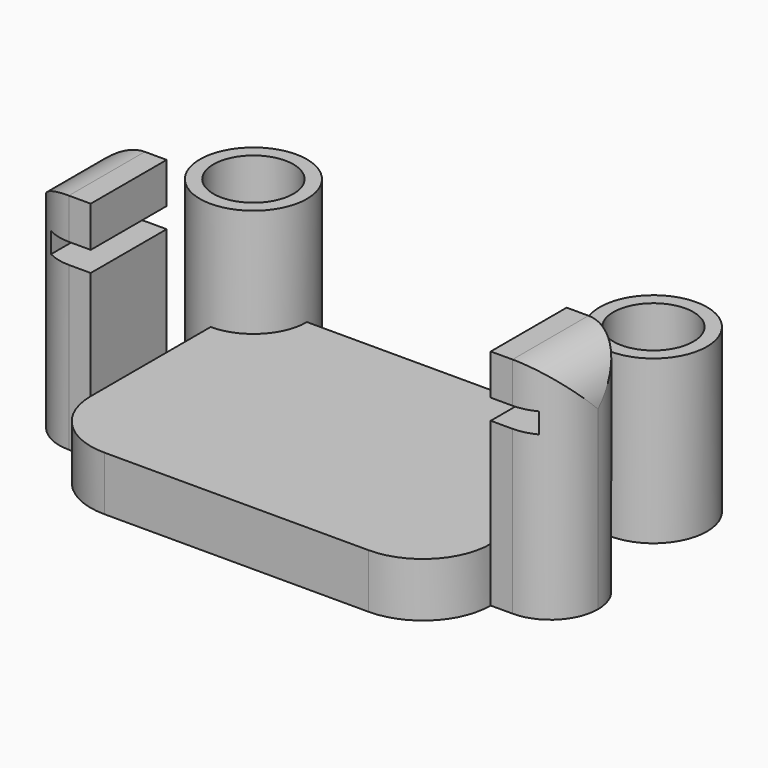
from build123d import *

# Parameters (mm, degrees)
F0_R         = 3.95
F0_R_2       = 2.95
F1_DEPTH     = 12
F3_DEPTH     = 4
F5_R         = 5
F6_W         = 3
F6_H         = 7
F6_W_2       = 2.1112600537
F7_DEPTH     = 16.5
F8_W         = 3.25
F8_H         = 1.5
F9_DEPTH     = 7
F10_T1_DEPTH = 34
F10_T3_DEPTH = 24.5


# Not quite as in the source:
# - a fillet or chamfer that OpenCascade refuses, or shapes differently, is made with other operations: its cross-section is extruded or revolved along the edge and cut away or added


with BuildPart() as f1:
    # F0 (on Top) → F1 (new body)
    with BuildSketch(Plane.XY):
        Circle(F0_R)
        Circle(F0_R_2, mode=Mode.SUBTRACT)
    extrude(amount=F1_DEPTH)


with BuildPart() as f1b:
    # F0 (on Top) → F1, piece 2 (new body)
    with BuildSketch(Plane.XY):
        with Locations((29.5, 0)):
            Circle(F0_R)
        with Locations((29.5, 0)):
            Circle(F0_R_2, mode=Mode.SUBTRACT)
    extrude(amount=F1_DEPTH)


with BuildPart() as f3:
    # F2 (on face) → F3 (new body)
    with BuildSketch(Plane(origin=(0, 0, 0), x_dir=(1, 0, 0), z_dir=(0, 0, -1))):
        with BuildLine():
            ThreePointArc((0, 3.95), (2.7930717857, 2.7930717857), (3.95, 0))
            Line((3.95, 0), (25.55, 0))
            ThreePointArc((25.55, 0), (26.7069282143, 2.7930717857), (29.5, 3.95))
            Line((29.5, 3.95), (29.5, 20))
            Line((29.5, 20), (0, 20))
            Line((0, 20), (0, 3.95))
        make_face()
    extrude(amount=-F3_DEPTH)

    # F4: union F1, F1b
    add(f1.part)
    add(f1b.part)

    # F5
    f5_edges = [f3.edges().sort_by_distance(p)[0] for p in [
        (0, -20, 2),
        (29.5, -20, 2),
    ]]
    fillet(f5_edges, radius=F5_R)

    # F6 (on face) → F7 (join)
    with BuildSketch(Plane(origin=(0, 0, 0), x_dir=(1, 0, 0), z_dir=(0, 0, -1))):
        with Locations((-3.6112600537, 11.5)):
            Rectangle(F6_W, F6_H)
        with Locations((-1.0556300269, 11.5)):
            Rectangle(F6_W_2, F6_H)
        with Locations((30.5556300269, 11.5)):
            Rectangle(F6_W_2, F6_H)
        with Locations((33.1112600537, 11.5)):
            Rectangle(F6_W, F6_H)
    extrude(amount=-F7_DEPTH)

    # F8 (on face) → F9 (cut, through all)
    with BuildSketch(Plane.XZ.offset(15)):
        with Locations((-1.625, 12.75)):
            Rectangle(F8_W, F8_H)
        with Locations((31.125, 12.75)):
            Rectangle(F8_W, F8_H)
    extrude(amount=-F9_DEPTH, mode=Mode.SUBTRACT)

    # F10: fillet of radius 3.5 on 6 edges, made by hand

    # F10_s2 → F10_t1 (cut)
    with BuildSketch(Plane.XY.offset(-8.75)):
        with BuildLine():
            ThreePointArc((-1.6112600537, -15), (-4.0861337879, -13.9748737342), (-5.1112600537, -11.5))
            Line((-5.1112600537, -11.5), (-5.1112600537, -15))
            Line((-5.1112600537, -15), (-1.6112600537, -15))
        make_face()
        with BuildLine():
            ThreePointArc((-5.1112600537, -11.5), (-4.0861337879, -9.0251262658), (-1.6112600537, -8))
            Line((-1.6112600537, -8), (-5.1112600537, -8))
            Line((-5.1112600537, -8), (-5.1112600537, -11.5))
        make_face()
        with BuildLine():
            ThreePointArc((34.6112600537, -11.5), (33.5861337879, -13.9748737342), (31.1112600537, -15))
            Line((31.1112600537, -15), (34.6112600537, -15))
            Line((34.6112600537, -15), (34.6112600537, -11.5))
        make_face()
        with BuildLine():
            ThreePointArc((31.1112600537, -8), (33.5861337879, -9.0251262658), (34.6112600537, -11.5))
            Line((34.6112600537, -11.5), (34.6112600537, -8))
            Line((34.6112600537, -8), (31.1112600537, -8))
        make_face()
    extrude(amount=F10_T1_DEPTH, mode=Mode.SUBTRACT)

    # F10_s4 → F10_t3 (cut)
    with BuildSketch(Plane.XZ.offset(-0.75)):
        with BuildLine():
            ThreePointArc((34.6112600537, 13), (33.5861337879, 15.4748737342), (31.1112600537, 16.5))
            Line((31.1112600537, 16.5), (34.6112600537, 16.5))
            Line((34.6112600537, 16.5), (34.6112600537, 13))
        make_face()
        with BuildLine():
            ThreePointArc((-5.1112600537, 13), (-4.0861337879, 15.4748737342), (-1.6112600537, 16.5))
            Line((-1.6112600537, 16.5), (-5.1112600537, 16.5))
            Line((-5.1112600537, 16.5), (-5.1112600537, 13))
        make_face()
    extrude(amount=F10_T3_DEPTH, mode=Mode.SUBTRACT)


solid = f3.part
